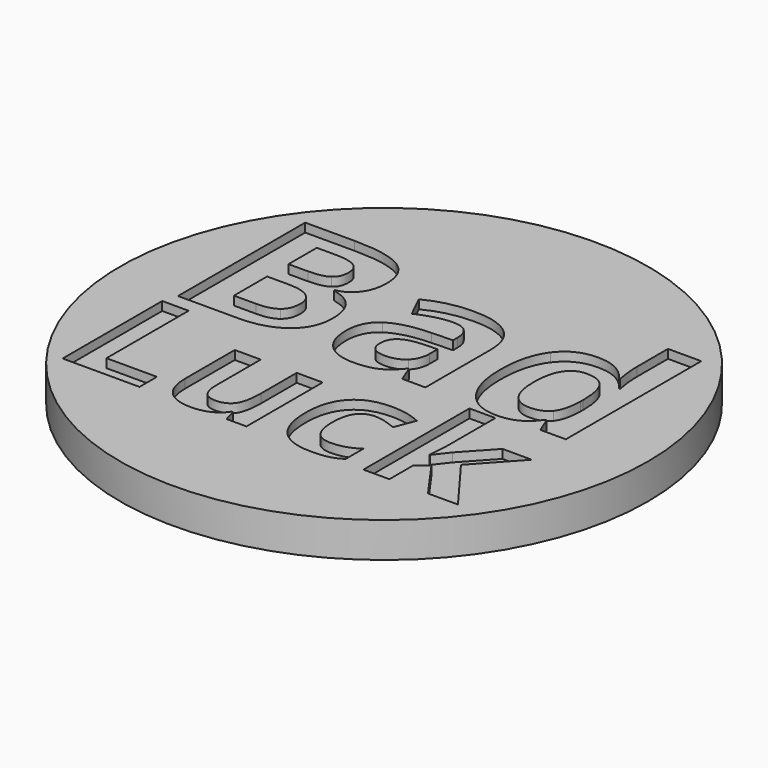
from build123d import *

# Parameters (mm, degrees)
F0_R         = 15
F1_DEPTH     = 2
F2_W         = 1.8908851162
F2_H         = 0.5043678919
F2_TEXT_SIZE = 9.9115957927
F3_DEPTH     = 0.5


# Not quite as in the source:
# - Text() gives the source's letters only with a copy of the font that has no kerning and outlines rounded to 1/6400 em; it was checked with that copy


with BuildPart() as f1:
    # F0 (on Top) → F1 (new body)
    with BuildSketch(Plane.XY):
        Circle(F0_R)
    extrude(amount=F1_DEPTH)

    # F2 (on face) → F3 (cut)
    with BuildSketch(Plane.XY.offset(2)):
        with Locations((9.8745163275, 8.7521839459)):
            Rectangle(F2_W, F2_H)
        with BuildLine():
            Line((10.8199588856, 8.5), (8.9290737694, 8.5))
            Line((8.9290737694, 8.5), (8.9290737694, 6.7910829075))
            add(Edge.make_bspline(
                [(9.0714835271, 5.4124773364), (8.9290737694, 6.1858414373), (8.9290737694, 6.7910829075)],
                knots=[0, 0, 0, 1, 1, 1], degree=2))
            Line((9.0714835271, 5.4124773364), (9.0101682147, 5.4124773364))
            add(Edge.make_bspline(
                [(7.0184095202, 6.4251689468), (8.3238322991, 6.4251689468), (9.0101682147, 5.4124773364)],
                knots=[0, 0, 0, 1, 1, 1], degree=2))
            add(Edge.make_bspline(
                [(5.0691759616, 5.4767595187), (5.7762799668, 6.4251689468), (7.0184095202, 6.4251689468)],
                knots=[0, 0, 0, 1, 1, 1], degree=2))
            add(Edge.make_bspline(
                [(4.3620719563, 2.8293225647), (4.3620719563, 4.5283500907), (5.0691759616, 5.4767595187)],
                knots=[0, 0, 0, 1, 1, 1], degree=2))
            add(Edge.make_bspline(
                [(5.0573084818, 0.2075984836), (4.3620719563, 1.1540299984), (4.3620719563, 2.8293225647)],
                knots=[0, 0, 0, 1, 1, 1], degree=2))
            add(Edge.make_bspline(
                [(6.9689616876, -0.7388330312), (5.7525450072, -0.7388330312), (5.0573084818, 0.2075984836)],
                knots=[0, 0, 0, 1, 1, 1], degree=2))
            add(Edge.make_bspline(
                [(8.9290737694, 0.2817702324), (8.2862519464, -0.7388330312), (6.9689616876, -0.7388330312)],
                knots=[0, 0, 0, 1, 1, 1], degree=2))
            Line((8.9290737694, 0.2817702324), (9.0101682147, 0.2817702324))
            Line((9.0101682147, 0.2817702324), (9.3741042622, -0.6142244932))
            Line((9.3741042622, -0.6142244932), (10.8199588856, -0.6142244932))
            Line((10.8199588856, -0.6142244932), (10.8199588856, 8.5))
        make_face()
        with BuildLine():
            add(Edge.make_bspline(
                [(7.6315626436, 0.764381078), (8.3535009987, 0.764381078), (8.6907352166, 1.1846876545)],
                knots=[0, 0, 0, 1, 1, 1], degree=2))
            add(Edge.make_bspline(
                [(6.6228268599, 1.2746827097), (6.9748954275, 0.764381078), (7.6315626436, 0.764381078)],
                knots=[0, 0, 0, 1, 1, 1], degree=2))
            add(Edge.make_bspline(
                [(6.2707582922, 2.8036096918), (6.2707582922, 1.7849843415), (6.6228268599, 1.2746827097)],
                knots=[0, 0, 0, 1, 1, 1], degree=2))
            add(Edge.make_bspline(
                [(6.6198599899, 4.3582495467), (6.2707582922, 3.8242129553), (6.2707582922, 2.8036096918)],
                knots=[0, 0, 0, 1, 1, 1], degree=2))
            add(Edge.make_bspline(
                [(7.5999160308, 4.8922861381), (6.9689616876, 4.8922861381), (6.6198599899, 4.3582495467)],
                knots=[0, 0, 0, 1, 1, 1], degree=2))
            add(Edge.make_bspline(
                [(8.7164480895, 4.4106642492), (8.3732801317, 4.8922861381), (7.5999160308, 4.8922861381)],
                knots=[0, 0, 0, 1, 1, 1], degree=2))
            add(Edge.make_bspline(
                [(9.0596160473, 2.8154771716), (9.0596160473, 3.9290423603), (8.7164480895, 4.4106642492)],
                knots=[0, 0, 0, 1, 1, 1], degree=2))
            Line((9.0596160473, 2.8154771716), (9.0596160473, 2.6117521015))
            add(Edge.make_bspline(
                [(8.6907352166, 1.1846876545), (9.0279694345, 1.6049942311), (9.0596160473, 2.6117521015)],
                knots=[0, 0, 0, 1, 1, 1], degree=2))
        make_face(mode=Mode.SUBTRACT)
        with BuildLine():
            Line((-8.4093142313, 8.4228613812), (-11.221906946, 8.4228613812))
            Line((-11.221906946, 8.4228613812), (-11.221906946, -0.6142244932))
            Line((-11.221906946, -0.6142244932), (-7.8416531138, -0.6142244932))
            add(Edge.make_bspline(
                [(-5.4147534929, 0.0780451624), (-6.3087703051, -0.6142244932), (-7.8416531138, -0.6142244932)],
                knots=[0, 0, 0, 1, 1, 1], degree=2))
            add(Edge.make_bspline(
                [(-4.5207366806, 2.0065106313), (-4.5207366806, 0.7703148179), (-5.4147534929, 0.0780451624)],
                knots=[0, 0, 0, 1, 1, 1], degree=2))
            add(Edge.make_bspline(
                [(-4.9014849911, 3.4039063788), (-4.5207366806, 2.8787703972), (-4.5207366806, 2.0065106313)],
                knots=[0, 0, 0, 1, 1, 1], degree=2))
            add(Edge.make_bspline(
                [(-6.1406476745, 4.1208999506), (-5.2822333017, 3.9290423603), (-4.9014849911, 3.4039063788)],
                knots=[0, 0, 0, 1, 1, 1], degree=2))
            Line((-6.1406476745, 4.1208999506), (-6.1406476745, 4.1822152629))
            add(Edge.make_bspline(
                [(-5.1299339774, 4.8062469095), (-5.5096933313, 4.2870446679), (-6.1406476745, 4.1822152629)],
                knots=[0, 0, 0, 1, 1, 1], degree=2))
            add(Edge.make_bspline(
                [(-4.7501746236, 6.1363936047), (-4.7501746236, 5.3254491511), (-5.1299339774, 4.8062469095)],
                knots=[0, 0, 0, 1, 1, 1], degree=2))
            add(Edge.make_bspline(
                [(-5.6184785629, 7.8759683534), (-4.7501746236, 7.3290753255), (-4.7501746236, 6.1363936047)],
                knots=[0, 0, 0, 1, 1, 1], degree=2))
            add(Edge.make_bspline(
                [(-8.4093142313, 8.4228613812), (-6.4867825023, 8.4228613812), (-5.6184785629, 7.8759683534)],
                knots=[0, 0, 0, 1, 1, 1], degree=2))
        make_face()
        with BuildLine():
            Line((-9.3053089568, 0.968106148), (-9.3053089568, 3.3238008901))
            Line((-9.3053089568, 3.3238008901), (-8.118560976, 3.3238008901))
            add(Edge.make_bspline(
                [(-6.5124953752, 2.1983682215), (-6.5124953752, 3.3238008901), (-8.118560976, 3.3238008901)],
                knots=[0, 0, 0, 1, 1, 1], degree=2))
            add(Edge.make_bspline(
                [(-6.8892878591, 1.2707268831), (-6.5124953752, 1.5733476183), (-6.5124953752, 2.1983682215)],
                knots=[0, 0, 0, 1, 1, 1], degree=2))
            add(Edge.make_bspline(
                [(-8.0572456636, 0.968106148), (-7.266080343, 0.968106148), (-6.8892878591, 1.2707268831)],
                knots=[0, 0, 0, 1, 1, 1], degree=2))
            Line((-8.0572456636, 0.968106148), (-9.3053089568, 0.968106148))
        make_face(mode=Mode.SUBTRACT)
        with BuildLine():
            Line((-8.1937216814, 4.8428383056), (-9.3053089568, 4.8428383056))
            Line((-9.3053089568, 4.8428383056), (-9.3053089568, 6.8523982199))
            Line((-9.3053089568, 6.8523982199), (-8.2985510864, 6.8523982199))
            add(Edge.make_bspline(
                [(-7.0959797991, 6.6269161035), (-7.475739153, 6.8523982199), (-8.2985510864, 6.8523982199)],
                knots=[0, 0, 0, 1, 1, 1], degree=2))
            add(Edge.make_bspline(
                [(-6.7162204452, 5.8812427889), (-6.7162204452, 6.4014339871), (-7.0959797991, 6.6269161035)],
                knots=[0, 0, 0, 1, 1, 1], degree=2))
            add(Edge.make_bspline(
                [(-7.0653221429, 5.0841437284), (-6.7162204452, 5.3254491511), (-6.7162204452, 5.8812427889)],
                knots=[0, 0, 0, 1, 1, 1], degree=2))
            add(Edge.make_bspline(
                [(-8.1937216814, 4.8428383056), (-7.4144238406, 4.8428383056), (-7.0653221429, 5.0841437284)],
                knots=[0, 0, 0, 1, 1, 1], degree=2))
        make_face(mode=Mode.SUBTRACT)
        with BuildLine():
            Line((1.1578524079, 0.325284325), (1.5237663687, -0.6142244932))
            Line((1.5237663687, -0.6142244932), (2.8390787142, -0.6142244932))
            Line((2.8390787142, -0.6142244932), (2.8390787142, 3.9903576727))
            add(Edge.make_bspline(
                [(2.0973612261, 5.832783913), (2.8390787142, 5.2265534861), (2.8390787142, 3.9903576727)],
                knots=[0, 0, 0, 1, 1, 1], degree=2))
            add(Edge.make_bspline(
                [(-0.0348293129, 6.4390143399), (1.3556437381, 6.4390143399), (2.0973612261, 5.832783913)],
                knots=[0, 0, 0, 1, 1, 1], degree=2))
            add(Edge.make_bspline(
                [(-2.6792993969, 5.8139937366), (-1.4866176761, 6.4390143399), (-0.0348293129, 6.4390143399)],
                knots=[0, 0, 0, 1, 1, 1], degree=2))
            Line((-2.6792993969, 5.8139937366), (-2.056256707, 4.5402175705))
            add(Edge.make_bspline(
                [(-0.108012105, 5.0406296357), (-0.9367577783, 5.0406296357), (-2.056256707, 4.5402175705)],
                knots=[0, 0, 0, 1, 1, 1], degree=2))
            add(Edge.make_bspline(
                [(0.967972731, 3.9903576727), (0.967972731, 5.0406296357), (-0.108012105, 5.0406296357)],
                knots=[0, 0, 0, 1, 1, 1], degree=2))
            Line((0.967972731, 3.9903576727), (0.967972731, 3.6877369375))
            Line((0.967972731, 3.6877369375), (-0.232620643, 3.6501565848))
            add(Edge.make_bspline(
                [(-2.5527129456, 3.0726059008), (-1.7833046714, 3.5947750124), (-0.232620643, 3.6501565848)],
                knots=[0, 0, 0, 1, 1, 1], degree=2))
            add(Edge.make_bspline(
                [(-3.3221212199, 1.4507169936), (-3.3221212199, 2.5504367892), (-2.5527129456, 3.0726059008)],
                knots=[0, 0, 0, 1, 1, 1], degree=2))
            add(Edge.make_bspline(
                [(-2.7505042758, -0.1691940003), (-3.3221212199, 0.4004450305), (-3.3221212199, 1.4507169936)],
                knots=[0, 0, 0, 1, 1, 1], degree=2))
            add(Edge.make_bspline(
                [(-1.183996941, -0.7388330312), (-2.1788873317, -0.7388330312), (-2.7505042758, -0.1691940003)],
                knots=[0, 0, 0, 1, 1, 1], degree=2))
            add(Edge.make_bspline(
                [(0.1293374912, -0.5064282182), (-0.3750304007, -0.7388330312), (-1.183996941, -0.7388330312)],
                knots=[0, 0, 0, 1, 1, 1], degree=2))
            add(Edge.make_bspline(
                [(1.1084045754, 0.325284325), (0.633705383, -0.2740234053), (0.1293374912, -0.5064282182)],
                knots=[0, 0, 0, 1, 1, 1], degree=2))
            Line((1.1084045754, 0.325284325), (1.1578524079, 0.325284325))
        make_face()
        with BuildLine():
            Line((0.2381227227, 2.562304269), (0.967972731, 2.5880171419))
            Line((0.967972731, 2.5880171419), (0.967972731, 2.0183781111))
            add(Edge.make_bspline(
                [(0.5753569406, 1.0175539806), (0.967972731, 1.3953354211), (0.967972731, 2.0183781111)],
                knots=[0, 0, 0, 1, 1, 1], degree=2))
            add(Edge.make_bspline(
                [(-0.4739260658, 0.63977254), (0.1827411503, 0.63977254), (0.5753569406, 1.0175539806)],
                knots=[0, 0, 0, 1, 1, 1], degree=2))
            add(Edge.make_bspline(
                [(-1.3877220111, 1.4388495138), (-1.3877220111, 0.63977254), (-0.4739260658, 0.63977254)],
                knots=[0, 0, 0, 1, 1, 1], degree=2))
            add(Edge.make_bspline(
                [(-0.9862056109, 2.2666062304), (-1.3877220111, 1.9946431515), (-1.3877220111, 1.4388495138)],
                knots=[0, 0, 0, 1, 1, 1], degree=2))
            add(Edge.make_bspline(
                [(0.2381227227, 2.562304269), (-0.5846892107, 2.5385693094), (-0.9862056109, 2.2666062304)],
                knots=[0, 0, 0, 1, 1, 1], degree=2))
        make_face(mode=Mode.SUBTRACT)
        with Locations((-12.3592070943, -8.5)):
            Text('Luck', F2_TEXT_SIZE, font='Open Sans', font_style=FontStyle.BOLD, text_align=(TextAlign.LEFT, TextAlign.BOTTOM))
    extrude(amount=-F3_DEPTH, mode=Mode.SUBTRACT)


solid = f1.part
